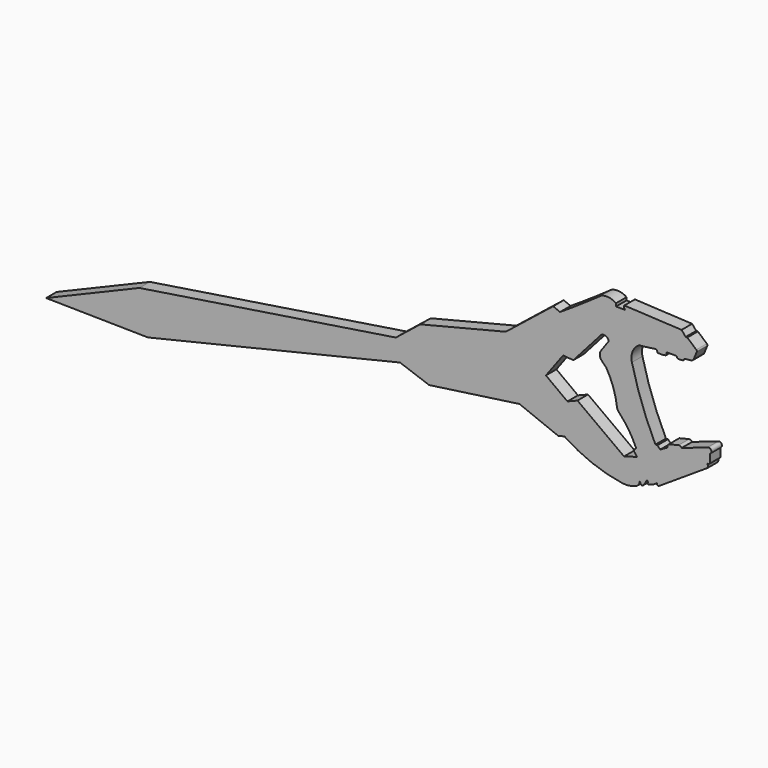
from build123d import *

# Parameters (mm, degrees)
F1_DEPTH = 5.08


# Not quite as in the source:
# - ends of sketch curves that miss each other by under 0.0002 mm in the source are joined


with BuildPart() as f1:
    # F0 (on Front) → F1 (new body)
    with BuildSketch(Plane.XZ):
        with BuildLine():
            Line((122.3705169674, 43.6478478759), (100.4099901217, 44.7520101639))
            ThreePointArc((100.4099901217, 44.7520101639), (100.0915452408, 44.5649170993), (100.1369538552, 44.1983805872))
            Line((100.1369538552, 44.1983805872), (100.4933528952, 43.3469744222))
            Line((100.4933528952, 43.3469744222), (97.0679359779, 43.3469744222))
            ThreePointArc((97.0679359779, 43.3469744222), (97.1316973251, 43.9112769391), (97.0679359779, 44.4755794561))
            ThreePointArc((97.0679359779, 44.4755794561), (94.352164437, 45.5363400819), (91.4515092493, 45.2416747635))
            ThreePointArc((91.4515092493, 45.2416747635), (83.5169492087, 39.7690696601), (75.469607442, 34.4637006676))
            Line((75.469607442, 34.4637006676), (72.8059848223, 35.5506727573))
            Line((72.8059848223, 35.5506727573), (54.5259908631, 20.9512186051))
            Line((54.5259908631, 20.9512186051), (21.5238705481, 12.7313591723))
            Line((21.5238705481, 12.7313591723), (12.1287463537, 5.188944246))
            Line((12.1287463537, 5.188944246), (-86.8316226794, -10.1466157916))
            Line((-86.8316226794, -10.1466157916), (-122.8382140398, -25.2789985389))
            Line((-122.8382140398, -25.2789985389), (-83.5318863392, -25.8913505822))
            Line((-83.5318863392, -25.8913505822), (13.7389805729, -2.7855467746))
            Line((13.7389805729, -2.7855467746), (24.9590244256, -6.7754736037))
            Line((24.9590244256, -6.7754736037), (59.8014198344, -1.8680947637))
            Line((59.8014198344, -1.8680947637), (74.7804443647, -7.8362995921))
            Line((74.7804443647, -7.8362995921), (77.1637969914, -7.2426764133))
            ThreePointArc((77.1637969914, -7.2426764133), (87.7830978003, -12.7533844887), (99.34301444, -15.8365290594))
            ThreePointArc((99.34301444, -15.8365290594), (102.2935896026, -15.8090472805), (105.1187411592, -14.9574794792))
            ThreePointArc((105.1187411592, -14.9574794792), (105.899310207, -14.1060464291), (106.1757861101, -12.9845357079))
            Line((106.1757861101, -12.9845357079), (106.7682035421, -14.0309760573))
            ThreePointArc((106.7682035421, -14.0309760573), (107.1058211072, -14.2278082292), (107.4434386724, -14.0309760573))
            ThreePointArc((107.4434386724, -14.0309760573), (108.2763784739, -13.0200234045), (108.8199970928, -11.8282630359))
            ThreePointArc((108.8199970928, -11.8282630359), (109.2695277638, -12.0590826755), (109.3121668662, -12.562607687))
            ThreePointArc((109.3121668662, -12.562607687), (109.3974608172, -12.9490474891), (109.7808973473, -13.0469617679))
            ThreePointArc((109.7808973473, -13.0469617679), (111.3986393651, -12.4328774082), (112.8510778468, -11.4923396397))
            ThreePointArc((112.8510778468, -11.4923396397), (113.1573925131, -12.1883188801), (113.9052785257, -12.0509060352))
            Line((113.9052785257, -12.0509060352), (132.3935237104, 0))
            ThreePointArc((132.3935237104, 0), (132.4837449873, 0.8029846441), (132.338838949, 1.5979226652))
            ThreePointArc((132.338838949, 1.5979226652), (133.0482342221, 1.5833492596), (133.4072056247, 2.1953897564))
            Line((133.4072056247, 2.1953897564), (133.4072056247, 5.2268817127))
            ThreePointArc((133.4072056247, 5.2268817127), (133.6969073142, 6.6313363292), (132.2924526977, 6.9210380187))
            Line((132.2924526977, 6.9210380187), (122.3704141488, 3.5393718949))
            ThreePointArc((122.3704141488, 3.5393718949), (121.873706248, 4.0268683816), (121.1812593401, 4.096788644))
            Line((121.1812593401, 4.096788644), (117.4436091822, 3.1937307858))
            ThreePointArc((117.4436091822, 3.1937307858), (117.0266780243, 2.6505498353), (117.0476117867, 1.966123862))
            Line((117.0476117867, 1.966123862), (114.1193957515, 0.3182646199))
            Line((114.1193957515, 0.3182646199), (113.0366831493, 1.4009768977))
            Line((113.0366831493, 1.4009768977), (112.2633179935, 1.4009768977))
            ThreePointArc((112.2633179935, 1.4009768977), (107.0399689979, 13.6404694995), (103.2035150013, 26.3829250952))
            ThreePointArc((103.2035150013, 26.3829250952), (103.4910499167, 30.2221985041), (106.029088113, 33.1172043332))
            ThreePointArc((106.029088113, 33.1172043332), (109.2898552798, 33.4516431179), (112.5333359919, 33.9252301607))
            ThreePointArc((112.5333359919, 33.9252301607), (112.8589818565, 33.5520971563), (112.9913329797, 33.074858591))
            ThreePointArc((112.9913329797, 33.074858591), (113.0214742771, 32.9498651341), (113.1128615921, 32.8594205615))
            ThreePointArc((113.1128615921, 32.8594205615), (114.605495502, 32.7922614875), (116.0903229782, 32.9588558937))
            ThreePointArc((116.0903229782, 32.9588558937), (116.3029445973, 33.0127632591), (116.4383345302, 33.1853422934))
            ThreePointArc((116.4383345302, 33.1853422934), (116.4779468759, 33.679151188), (116.554347608, 34.1686195634))
            Line((116.554347608, 34.1686195634), (119.7698420306, 34.1686195634))
            ThreePointArc((119.7698420306, 34.1686195634), (120.3377346413, 34.0985961328), (120.6763827811, 33.6373773826))
            ThreePointArc((120.6763827811, 33.6373773826), (120.705556032, 33.5058788759), (120.7971017103, 33.4070743991))
            ThreePointArc((120.7971017103, 33.4070743991), (121.8693321552, 33.350668944), (122.933876584, 33.4906863059))
            ThreePointArc((122.933876584, 33.4906863059), (123.0810934781, 33.5938295086), (123.11967467, 33.7693938154))
            ThreePointArc((123.11967467, 33.7693938154), (123.4255269006, 34.1427273195), (123.8907699445, 34.2710721767))
            Line((123.8907699445, 34.2710721767), (125.9903685922, 34.462153965))
            ThreePointArc((125.9903685922, 34.462153965), (126.6924885264, 34.7530229594), (127.1051986302, 35.3911824568))
            Line((127.1051986302, 35.3911824568), (128.2572048943, 38.1039466219))
            ThreePointArc((128.2572048943, 38.1039466219), (128.2729126944, 38.4579608874), (128.0528186952, 38.7356864116))
            Line((128.0528186952, 38.7356864116), (124.5782394715, 41.7643239316))
            Line((124.5782394715, 41.7643239316), (123.9465066021, 41.7643239316))
            Line((123.9465066021, 41.7643239316), (122.3705169674, 43.6478478759))
        make_face()
        with BuildLine():
            Line((70.0165052271, 11.150856785), (76.6579802489, 20.1397516237))
            Line((76.6579802489, 20.1397516237), (80.5816721076, 19.7545750625))
            Line((80.5816721076, 19.7545750625), (91.4935366546, 32.0359588494))
            ThreePointArc((91.4935366546, 32.0359588494), (93.1959095158, 32.0009597447), (94.2558714279, 30.6683761485))
            Line((94.2558714279, 30.6683761485), (91.2971296419, 26.5111941478))
            ThreePointArc((91.2971296419, 26.5111941478), (90.8112616397, 24.8754815968), (91.4297100848, 23.2851530817))
            Line((91.4297100848, 23.2851530817), (93.3299813237, 21.2964983411))
            ThreePointArc((93.3299813237, 21.2964983411), (96.0132194113, 15.5328655264), (97.4206326201, 9.3329931151))
            ThreePointArc((97.4206326201, 9.3329931151), (97.6181949936, 8.6221123526), (98.0063865531, 7.9946654121))
            ThreePointArc((98.0063865531, 7.9946654121), (101.9070751405, 3.1730744617), (104.8498501941, -2.2861549466))
            ThreePointArc((104.8498501941, -2.2861549466), (104.2291914062, -2.8435135125), (104.0495855612, -3.6581346774))
            Line((104.0495855612, -3.6581346774), (105.1997786885, -5.0801357056))
            Line((105.1997786885, -5.0801357056), (100.1594934993, -6.5642189378))
            Line((100.1594934993, -6.5642189378), (82.2009610937, 6.5729623924))
            Line((82.2009610937, 6.5729623924), (78.3157963351, 5.0188977865))
            Line((78.3157963351, 5.0188977865), (70.0165052271, 11.150856785))
        make_face(mode=Mode.SUBTRACT)
    extrude(amount=F1_DEPTH)


solid = f1.part
